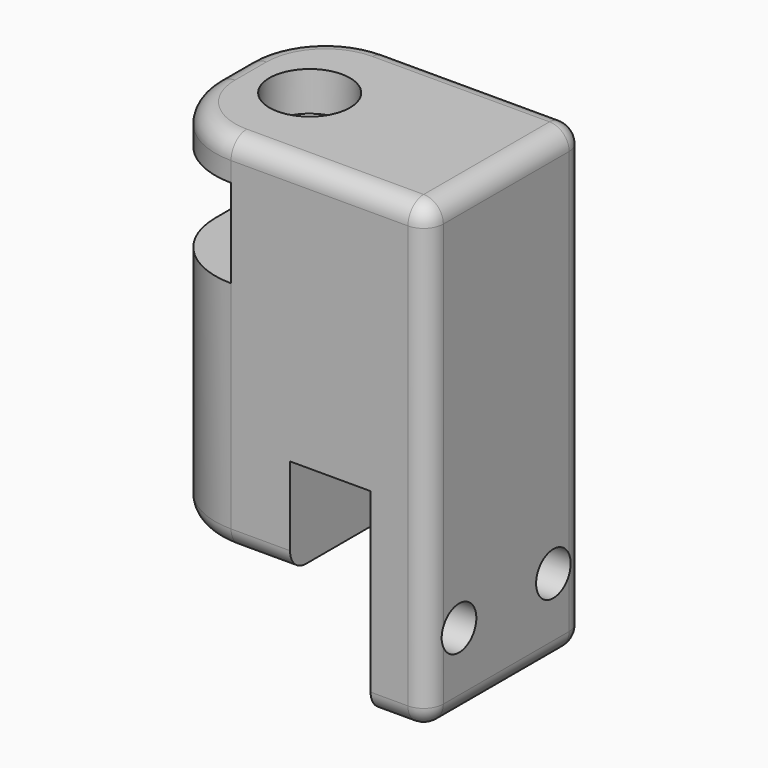
from build123d import *

# Parameters (mm, degrees)
F0_R          = 4.1
F1_DEPTH      = 34
F3_DEPTH      = 9
F4_R          = 4.1
F5_DEPTH      = 4
F6_W          = 8.2
F6_H          = 20
F7_DEPTH      = 20
F8_W          = 15.1884564608
F8_H          = 21.6641027853
F9_DEPTH      = 10
F10_R         = 2.2
F11_DEPTH     = 25
F12_T1_DEPTH  = 8.8
F12_T3_DEPTH  = 18
F12_T5_DEPTH  = 16
F12_T7_DEPTH  = 43
F12_T9_DEPTH  = 4
F12_T11_DEPTH = 11
F12_S15_W     = 2
F12_S15_H     = 2
F12_T16_DEPTH = 2
F12_S21_W     = 2
F12_S21_H     = 2
F12_T22_DEPTH = 2
F12_S27_W     = 2
F12_S27_H     = 2
F12_T28_DEPTH = 2
F12_S33_W     = 2
F12_S33_H     = 2
F12_T34_DEPTH = 2
F12_T38_ANGLE = 90
F12_T40_ANGLE = 90
F12_T42_ANGLE = 90
F12_T44_ANGLE = 90


# Not quite as in the source:
# - a fillet or chamfer that OpenCascade refuses, or shapes differently, is made with other operations: its cross-section is extruded or revolved along the edge and cut away or added


with BuildPart() as f1:
    # F0 (on Top) → F1 (new body)
    with BuildSketch(Plane.XY):
        with BuildLine():
            ThreePointArc((-8, -2), (-5.6568542495, -7.6568542495), (0, -10))
            Line((0, -10), (20, -10))
            Line((20, -10), (20, 10))
            Line((20, 10), (0, 10))
            ThreePointArc((0, 10), (-5.6568542495, 7.6568542495), (-8, 2))
            Line((-8, 2), (-8, -2))
        make_face()
        Circle(F0_R, mode=Mode.SUBTRACT)
    extrude(amount=F1_DEPTH)

    # F2 (on face) → F3 (join)
    with BuildSketch(Plane.XY.offset(34)):
        with BuildLine():
            Line((0, 10), (0, 8.5))
            ThreePointArc((0, 8.5), (8.5, 0), (0, -8.5))
            Line((0, -8.5), (0, -10))
            Line((0, -10), (20, -10))
            Line((20, -10), (20, 10))
            Line((20, 10), (0, 10))
        make_face()
    extrude(amount=F3_DEPTH)

    # F4 (on face) → F5 (join)
    with BuildSketch(Plane.XY.offset(43)):
        with BuildLine():
            Line((20, -10), (20, 10))
            Line((20, 10), (0, 10))
            ThreePointArc((0, 10), (-5.6568542495, 7.6568542495), (-8, 2))
            Line((-8, 2), (-8, -2))
            ThreePointArc((-8, -2), (-5.6568542495, -7.6568542495), (0, -10))
            Line((0, -10), (20, -10))
        make_face()
        Circle(F4_R, mode=Mode.SUBTRACT)
    extrude(amount=F5_DEPTH)

    # F6 (on face) → F7 (cut)
    with BuildSketch(Plane(origin=(0, 0, 0), x_dir=(1, 0, 0), z_dir=(0, 0, -1))):
        with Locations((10.1, 0)):
            Rectangle(F6_W, F6_H)
    extrude(amount=-F7_DEPTH, mode=Mode.SUBTRACT)

    # F8 (on face) → F9 (cut)
    with BuildSketch(Plane(origin=(0, 0, 0), x_dir=(1, 0, 0), z_dir=(0, 0, -1))):
        with Locations((-1.5942282304, 0.8320513926)):
            Rectangle(F8_W, F8_H)
    extrude(amount=-F9_DEPTH, mode=Mode.SUBTRACT)

    # F10 (on face) → F11 (cut)
    with BuildSketch(Plane(origin=(14.2, 0, 0), x_dir=(0, -1, 0), z_dir=(-1, 0, 0))):
        with Locations((6, 8)):
            Circle(F10_R)
        with Locations((-6, 8)):
            Circle(F10_R)
    extrude(amount=-F11_DEPTH, mode=Mode.SUBTRACT)

    # F12: fillet of radius 2 on 16 edges, made by hand

    # F12_s2 → F12_t1 (cut)
    with BuildSketch(Plane.YZ.offset(9.2)):
        with BuildLine():
            ThreePointArc((10, 2), (9.4142135624, 0.5857864376), (8, 0))
            Line((8, 0), (10, 0))
            Line((10, 0), (10, 2))
        make_face()
        with BuildLine():
            ThreePointArc((-10, 2), (-9.4142135624, 0.5857864376), (-8, 0))
            Line((-8, 0), (-10, 0))
            Line((-10, 0), (-10, 2))
        make_face()
    extrude(amount=F12_T1_DEPTH, mode=Mode.SUBTRACT)

    # F12_s4 → F12_t3 (cut)
    with BuildSketch(Plane.YZ):
        with BuildLine():
            ThreePointArc((10, 45), (9.4142135624, 46.4142135624), (8, 47))
            Line((8, 47), (10, 47))
            Line((10, 47), (10, 45))
        make_face()
        with BuildLine():
            ThreePointArc((-10, 45), (-9.4142135624, 46.4142135624), (-8, 47))
            Line((-8, 47), (-10, 47))
            Line((-10, 47), (-10, 45))
        make_face()
    extrude(amount=F12_T3_DEPTH, mode=Mode.SUBTRACT)

    # F12_s6 → F12_t5 (cut)
    with BuildSketch(Plane.XZ.offset(-8)):
        with BuildLine():
            ThreePointArc((20, 45), (19.4142135624, 46.4142135624), (18, 47))
            Line((18, 47), (20, 47))
            Line((20, 47), (20, 45))
        make_face()
        with BuildLine():
            ThreePointArc((20, 2), (19.4142135624, 0.5857864376), (18, 0))
            Line((18, 0), (20, 0))
            Line((20, 0), (20, 2))
        make_face()
    extrude(amount=F12_T5_DEPTH, mode=Mode.SUBTRACT)

    # F12_s8 → F12_t7 (cut)
    with BuildSketch(Plane.XY.offset(2)):
        with BuildLine():
            ThreePointArc((18, 10), (19.4142135624, 9.4142135624), (20, 8))
            Line((20, 8), (20, 10))
            Line((20, 10), (18, 10))
        make_face()
        with BuildLine():
            ThreePointArc((18, -10), (19.4142135624, -9.4142135624), (20, -8))
            Line((20, -8), (20, -10))
            Line((20, -10), (18, -10))
        make_face()
    extrude(amount=F12_T7_DEPTH, mode=Mode.SUBTRACT)

    # F12_s10 → F12_t9 (cut)
    with BuildSketch(Plane.XZ.offset(-2)):
        with BuildLine():
            ThreePointArc((-6, 10), (-7.4142135624, 10.5857864376), (-8, 12))
            Line((-8, 12), (-8, 10))
            Line((-8, 10), (-6, 10))
        make_face()
        with BuildLine():
            ThreePointArc((-6, 47), (-7.4142135624, 46.4142135624), (-8, 45))
            Line((-8, 45), (-8, 47))
            Line((-8, 47), (-6, 47))
        make_face()
    extrude(amount=F12_T9_DEPTH, mode=Mode.SUBTRACT)

    # F12_s12 → F12_t11 (cut)
    with BuildSketch(Plane.YZ):
        with BuildLine():
            ThreePointArc((-8, 10), (-9.4142135624, 10.5857864376), (-10, 12))
            Line((-10, 12), (-10, 10))
            Line((-10, 10), (-8, 10))
        make_face()
        with BuildLine():
            ThreePointArc((8, 10), (9.4142135624, 10.5857864376), (10, 12))
            Line((10, 12), (10, 10))
            Line((10, 10), (8, 10))
        make_face()
    extrude(amount=F12_T11_DEPTH, mode=Mode.SUBTRACT)


with BuildPart() as f12_tool14:
    # F12_s15 → F12_t16 (new body)
    with BuildSketch(Plane.YZ.offset(18)):
        with Locations((9, 1)):
            Rectangle(F12_S15_W, F12_S15_H)
    extrude(amount=F12_T16_DEPTH)

    # F12_s17 → F12_t18 (revolve, cut)
    with BuildSketch(Plane(origin=(18, 8, 2), x_dir=(0, -0.7071067812, 0.7071067812), z_dir=(0, 0.7071067812, 0.7071067812))):
        with BuildLine():
            ThreePointArc((0, -2), (2, 0), (0, 2))
            Line((0, 2), (0, -2))
        make_face()
    revolve(axis=Axis((18, 8, 2), (1, 0, 0)), mode=Mode.SUBTRACT)


with BuildPart() as f1_1:
    add(f1.part)

    # F12_t13: cut F12_tool14
    add(f12_tool14.part, mode=Mode.SUBTRACT)


with BuildPart() as f12_tool20:
    # F12_s21 → F12_t22 (new body)
    with BuildSketch(Plane.XY.offset(45)):
        with Locations((19, 9)):
            Rectangle(F12_S21_W, F12_S21_H)
    extrude(amount=F12_T22_DEPTH)

    # F12_s23 → F12_t24 (revolve, cut)
    with BuildSketch(Plane(origin=(18, 8, 45), x_dir=(-0.7071067812, -0.7071067812, 0), z_dir=(-0.7071067812, 0.7071067812, 0))):
        with BuildLine():
            ThreePointArc((0, -2), (2, 0), (0, 2))
            Line((0, 2), (0, -2))
        make_face()
    revolve(axis=Axis((18, 8, 45), (0, 0, 1)), mode=Mode.SUBTRACT)


with BuildPart() as f1_2:
    add(f1_1.part)

    # F12_t19: cut F12_tool20
    add(f12_tool20.part, mode=Mode.SUBTRACT)


with BuildPart() as f12_tool26:
    # F12_s27 → F12_t28 (new body)
    with BuildSketch(Plane.XY.offset(45)):
        with Locations((19, -9)):
            Rectangle(F12_S27_W, F12_S27_H)
    extrude(amount=F12_T28_DEPTH)

    # F12_s29 → F12_t30 (revolve, cut)
    with BuildSketch(Plane(origin=(18, -8, 45), x_dir=(-0.7071067812, 0.7071067812, 0), z_dir=(0.7071067812, 0.7071067812, 0))):
        with BuildLine():
            ThreePointArc((0, -2), (2, 0), (0, 2))
            Line((0, 2), (0, -2))
        make_face()
    revolve(axis=Axis((18, -8, 45), (0, 0, 1)), mode=Mode.SUBTRACT)


with BuildPart() as f1_3:
    add(f1_2.part)

    # F12_t25: cut F12_tool26
    add(f12_tool26.part, mode=Mode.SUBTRACT)


with BuildPart() as f12_tool32:
    # F12_s33 → F12_t34 (new body)
    with BuildSketch(Plane.YZ.offset(18)):
        with Locations((-9, 1)):
            Rectangle(F12_S33_W, F12_S33_H)
    extrude(amount=F12_T34_DEPTH)

    # F12_s35 → F12_t36 (revolve, cut)
    with BuildSketch(Plane(origin=(18, -8, 2), x_dir=(0, 0.7071067812, 0.7071067812), z_dir=(0, 0.7071067812, -0.7071067812))):
        with BuildLine():
            ThreePointArc((0, -2), (2, 0), (0, 2))
            Line((0, 2), (0, -2))
        make_face()
    revolve(axis=Axis((18, -8, 2), (1, 0, 0)), mode=Mode.SUBTRACT)


with BuildPart() as f1_4:
    add(f1_3.part)

    # F12_t31: cut F12_tool32
    add(f12_tool32.part, mode=Mode.SUBTRACT)

    # F12_s37 → F12_t38 (revolve, cut)
    with BuildSketch(Plane.YZ):
        with BuildLine():
            ThreePointArc((-8, 10), (-9.4142135624, 10.5857864376), (-10, 12))
            Line((-10, 12), (-10, 10))
            Line((-10, 10), (-8, 10))
        make_face()
    revolve(axis=Axis((0, -2, 10), (0, 0, -1)), revolution_arc=F12_T38_ANGLE, mode=Mode.SUBTRACT)

    # F12_s39 → F12_t40 (revolve, cut)
    with BuildSketch(Plane.XZ.offset(-2)):
        with BuildLine():
            ThreePointArc((-8, 12), (-7.4142135624, 10.5857864376), (-6, 10))
            Line((-6, 10), (-8, 10))
            Line((-8, 10), (-8, 12))
        make_face()
    revolve(axis=Axis((0, 2, 10), (0, 0, -1)), revolution_arc=F12_T40_ANGLE, mode=Mode.SUBTRACT)

    # F12_s41 → F12_t42 (revolve, cut)
    with BuildSketch(Plane.YZ):
        with BuildLine():
            ThreePointArc((10, 45), (9.4142135624, 46.4142135624), (8, 47))
            Line((8, 47), (10, 47))
            Line((10, 47), (10, 45))
        make_face()
    revolve(axis=Axis((0, 2, 47), (0, 0, 1)), revolution_arc=F12_T42_ANGLE, mode=Mode.SUBTRACT)

    # F12_s43 → F12_t44 (revolve, cut)
    with BuildSketch(Plane.XZ.offset(2)):
        with BuildLine():
            ThreePointArc((-6, 47), (-7.4142135624, 46.4142135624), (-8, 45))
            Line((-8, 45), (-8, 47))
            Line((-8, 47), (-6, 47))
        make_face()
    revolve(axis=Axis((0, -2, 47), (0, 0, 1)), revolution_arc=F12_T44_ANGLE, mode=Mode.SUBTRACT)


solid = f1_4.part
